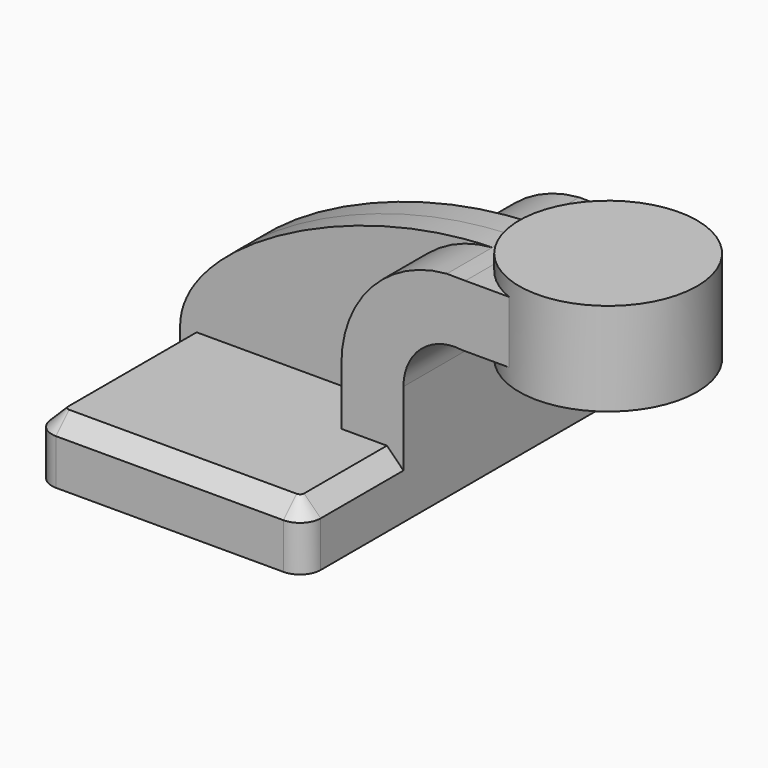
from build123d import *

# Parameters (mm, degrees)
F1_DEPTH     = 63.5
F0_W         = 23.4752528609
F0_H         = 19.05
F2_DEPTH     = 25.4
F3_DEPTH     = 7.9375
F5_R         = 6.35
F6_T1_DEPTH  = 69.85
F6_T3_DEPTH  = 31.75
F6_T5_DEPTH  = 31.75
F6_T7_DEPTH  = 49.2125
F6_T9_DEPTH  = 49.2125
F6_T12_ANGLE = 90
F6_T14_ANGLE = 90
F6_T16_ANGLE = 90
F6_T18_ANGLE = 90


# Not quite as in the source:
# - a fillet or chamfer that OpenCascade refuses, or shapes differently, is made with other operations: its cross-section is extruded or revolved along the edge and cut away or added


with BuildPart() as f1:
    # F0 (on Front) → F1 (new body, symmetric)
    with BuildSketch(Plane.XZ):
        Polygon((41.275, -9.525), (41.275, 9.525), (22.225, 9.525), (-41.275, 9.525), (-41.275, -9.525), align=None)
    extrude(amount=F1_DEPTH, both=True)

    # F0 (on Front) → F2 (join, symmetric)
    with BuildSketch(Plane.XZ):
        with BuildLine():
            Line((22.225, 9.525), (41.275, 9.525))
            Line((41.275, 9.525), (41.275, 27.1406874123))
            ThreePointArc((41.275, 27.1406874123), (46.6962412965, 39.0878441439), (59.257306012, 42.8752))
            Line((59.257306012, 42.8752), (60.325, 42.8752))
            Line((60.325, 42.8752), (60.325, 61.9252))
            Line((60.325, 61.9252), (60.2794263112, 61.9252))
            add(Edge.make_bspline(
                [(54.6017831222, 61.972601166), (56.5099245484, 62.0075695852), (58.404061726, 61.9925812099), (60.2794263112, 61.9252)],
                knots=[109.5395820666, 109.5395820666, 109.5395820666, 109.5395820666, 114.2763425362, 114.2763425362, 114.2763425362, 114.2763425362], degree=3))
            ThreePointArc((54.6017831222, 61.972601166), (31.5692249975, 50.9183991456), (22.225, 27.1406874123))
            Line((22.225, 27.1406874123), (22.225, 9.525))
        make_face()
        with Locations((72.0626264304, 52.4002)):
            Rectangle(F0_W, F0_H)
    extrude(amount=F2_DEPTH, both=True)

    # F0 (on Front) → F3 (join, symmetric)
    with BuildSketch(Plane.XZ):
        with BuildLine():
            Line((-41.275, 9.525), (22.225, 9.525))
            Line((22.225, 9.525), (22.225, 27.1406874123))
            ThreePointArc((22.225, 27.1406874123), (31.5692249975, 50.9183991456), (54.6017831222, 61.972601166))
            add(Edge.make_bspline(
                [(-41.275, 9.525), (-41.1406298822, 33.6391321553), (10.4752084943, 61.1639417355), (54.6017831222, 61.972601166)],
                knots=[0, 0, 0, 0, 109.5395820666, 109.5395820666, 109.5395820666, 109.5395820666], degree=3))
        make_face()
    extrude(amount=F3_DEPTH, both=True)

    # F0 (on Front) → F4 (revolve)
    with BuildSketch(Plane.XZ):
        Polygon((83.8002528609, 61.9252), (83.8002528609, 42.8752), (83.8002528609, 38.1), (111.125, 38.1), (111.125, 66.675), (83.8002528609, 66.675), align=None)
    revolve(axis=Axis((83.8002528609, 0, 52.3875), (0, 0, 1)))

    # F5
    f5_edges = [f1.edges().sort_by_distance(p)[0] for p in [
        (-41.275, -63.5, 0),
        (41.275, -63.5, 0),
        (41.275, 63.5, 0),
        (-41.275, 63.5, 0),
    ]]
    fillet(f5_edges, radius=F5_R)

    # F6: chamfer of 5.08 on 10 edges, made by hand

    # F6_s2 → F6_t1 (cut)
    with BuildSketch(Plane.YZ.offset(-34.925)):
        Polygon((-58.42, 9.525), (-63.5, 4.445), (-63.5, 9.525), align=None)
        Polygon((58.42, 9.525), (63.5, 4.445), (63.5, 9.525), align=None)
    extrude(amount=F6_T1_DEPTH, mode=Mode.SUBTRACT)

    # F6_s4 → F6_t3 (cut)
    with BuildSketch(Plane.XZ.offset(-57.15)):
        Polygon((41.275, 4.445), (36.195, 9.525), (41.275, 9.525), align=None)
    extrude(amount=F6_T3_DEPTH, mode=Mode.SUBTRACT)

    # F6_s6 → F6_t5 (cut)
    with BuildSketch(Plane.XZ.offset(25.4)):
        Polygon((41.275, 4.445), (36.195, 9.525), (41.275, 9.525), align=None)
    extrude(amount=F6_T5_DEPTH, mode=Mode.SUBTRACT)

    # F6_s8 → F6_t7 (cut)
    with BuildSketch(Plane.XZ.offset(-57.15)):
        Polygon((-36.195, 9.525), (-41.275, 4.445), (-41.275, 9.525), align=None)
    extrude(amount=F6_T7_DEPTH, mode=Mode.SUBTRACT)

    # F6_s10 → F6_t9 (cut)
    with BuildSketch(Plane.XZ.offset(7.9375)):
        Polygon((-36.195, 9.525), (-41.275, 4.445), (-41.275, 9.525), align=None)
    extrude(amount=F6_T9_DEPTH, mode=Mode.SUBTRACT)

    # F6_s11 → F6_t12 (revolve, cut)
    with BuildSketch(Plane.XZ.offset(-57.15)):
        Polygon((36.195, 9.525), (41.275, 4.445), (41.275, 9.525), align=None)
    revolve(axis=Axis((34.925, 57.15, 9.525), (0, 0, 1)), revolution_arc=F6_T12_ANGLE, mode=Mode.SUBTRACT)

    # F6_s13 → F6_t14 (revolve, cut)
    with BuildSketch(Plane.YZ.offset(-34.925)):
        Polygon((58.42, 9.525), (63.5, 4.445), (63.5, 9.525), align=None)
    revolve(axis=Axis((-34.925, 57.15, 9.525), (0, 0, 1)), revolution_arc=F6_T14_ANGLE, mode=Mode.SUBTRACT)

    # F6_s15 → F6_t16 (revolve, cut)
    with BuildSketch(Plane.XZ.offset(57.15)):
        Polygon((41.275, 4.445), (36.195, 9.525), (41.275, 9.525), align=None)
    revolve(axis=Axis((34.925, -57.15, 9.525), (0, 0, -1)), revolution_arc=F6_T16_ANGLE, mode=Mode.SUBTRACT)

    # F6_s17 → F6_t18 (revolve, cut)
    with BuildSketch(Plane.YZ.offset(-34.925)):
        Polygon((-58.42, 9.525), (-63.5, 4.445), (-63.5, 9.525), align=None)
    revolve(axis=Axis((-34.925, -57.15, 9.525), (0, 0, -1)), revolution_arc=F6_T18_ANGLE, mode=Mode.SUBTRACT)


solid = f1.part
